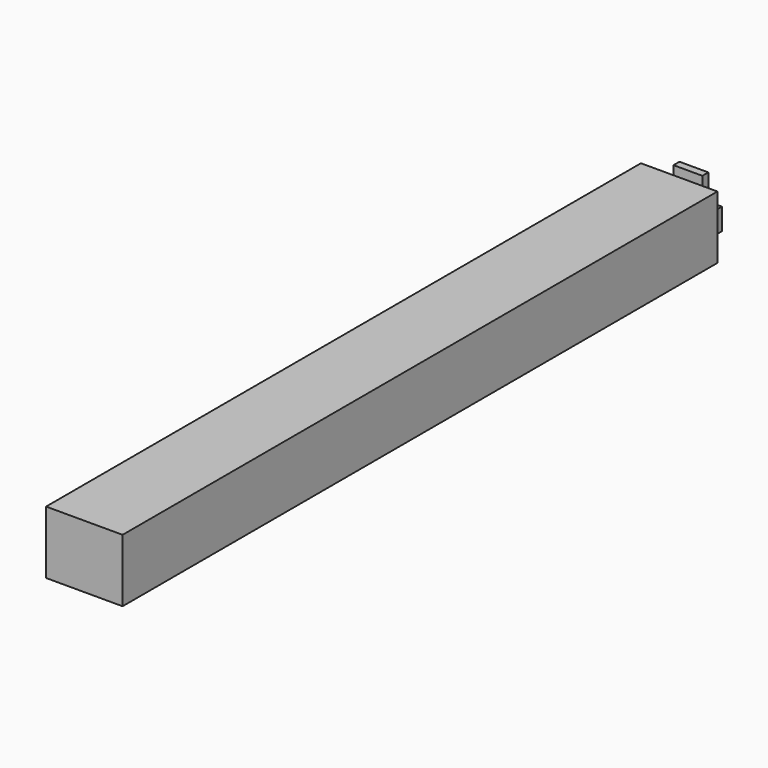
from build123d import *

# Parameters (mm, degrees)
F0_W      = 78.6321908236
F0_H      = 50.2420589328
F0_W_2    = 83.0053240061
F1_DEPTH  = 25.4
F2_W      = 26.6048051417
F2_H      = 12.7
F2_W_2    = 1.4717131853
F2_H_2    = 25.4
F3_DEPTH  = 25.4
F4_W      = 261.3360136747
F4_H      = 214.8963138461
F5_DEPTH  = 2540
F6_W      = 91.9215381145
F6_H      = 68.2068861365
F7_DEPTH  = 25.4
F8_W      = 18.1767717004
F8_H      = 111.8716299534
F8_H_2    = 16.7573786616
F9_DEPTH  = 25.4
F10_W     = 19.8279470205
F10_H     = 1.2968182564
F11_DEPTH = 25.4
F10_W_2   = 29.5902959347
F10_H_2   = 243.1764304638
F12_W     = 25.4
F12_H     = 71.0515528917
F13_DEPTH = 25.4
F14_W     = 21.7962116003
F14_H     = 10.9980255365
F15_DEPTH = 25.4
F16_W     = 95.2623337507
F16_H     = 72.595404768
F17_DEPTH = 25.4
F18_W     = 88.901007548
F18_H     = 12.7
F19_DEPTH = 25.4
F20_W     = 343.005374074
F20_H     = 14.3458449006
F21_DEPTH = 25.4
F22_W     = 127.9820352793
F22_H     = 85.2384865284
F23_DEPTH = 25.4
F24_W     = 127.9820352793
F24_H     = 73.9392116666
F25_DEPTH = 25.4


with BuildPart() as f1:
    # F0 (on Front) → F1 (new body)
    with BuildSketch(Plane.XZ):
        Polygon((-83.0053240061, 0), (0, 0), (78.6321908236, 0), (78.6321908236, 52.9869496822), (-83.0053240061, 52.9869496822), align=None)
        with Locations((39.3160954118, -25.1210294664)):
            Rectangle(F0_W, F0_H)
        with Locations((-41.502662003, -25.1210294664)):
            Rectangle(F0_W_2, F0_H)
    extrude(amount=F1_DEPTH)

    # F2 (on face) → F3 (join)
    with BuildSketch(Plane(origin=(0, 0, -50.2420589328), x_dir=(1, 0, 0), z_dir=(0, 0, -1))):
        Polygon((78.6321908236, 25.7508095026), (-56.4005188644, 25.7508095026), (-56.4005188644, 25.4), (77.1604776382, 25.4), (78.6321908236, 25.4), align=None)
        Polygon((77.1604776382, 25.4), (-56.4005188644, 25.4), (-56.4005188644, 12.7), (-56.4005188644, 0), (77.1604776382, 0), align=None)
        with Locations((-69.7029214352, 19.05)):
            Rectangle(F2_W, F2_H)
        with Locations((77.8963342309, 12.7)):
            Rectangle(F2_W_2, F2_H_2)
        with Locations((-69.7029214352, 6.35)):
            Rectangle(F2_W, F2_H)
    extrude(amount=F3_DEPTH)

    # F4 (on face) → F5 (join)
    with BuildSketch(Plane.XZ.offset(25.4)):
        with Locations((-6.4808502793, -16.0813815892)):
            Rectangle(F4_W, F4_H)
    extrude(amount=F5_DEPTH)

    # F16 (on face) → F17 (join)
    with BuildSketch(Plane(origin=(0, 0, -75.6420589328), x_dir=(1, 0, 0), z_dir=(0, 0, -1))):
        with Locations((-26.4344289899, -10.897702384)):
            Rectangle(F16_W, F16_H)
    extrude(amount=F17_DEPTH)


with BuildPart() as f7:
    # F6 (on face) → F7 (new body)
    with BuildSketch(Plane(origin=(-83.0053240061, 0, 0), x_dir=(0, -1, 0), z_dir=(-1, 0, 0))):
        with Locations((-45.9607690573, -41.5386158645)):
            Rectangle(F6_W, F6_H)
    extrude(amount=F7_DEPTH)


with BuildPart() as f9:
    # F8 (on face) → F9 (new body)
    with BuildSketch(Plane(origin=(-83.0053240061, 0, 0), x_dir=(0, -1, 0), z_dir=(-1, 0, 0))):
        with Locations((9.0883858502, -2.9488652945)):
            Rectangle(F8_W, F8_H)
        with Locations((9.0883858502, -67.263369602)):
            Rectangle(F8_W, F8_H_2)
        Polygon((18.1767717004, 52.9869496822), (18.1767717004, -58.8846802711), (18.1767717004, -75.6420589328), (25.4, -75.6420589328), (25.4, 52.9869496822), align=None)
    extrude(amount=F9_DEPTH)


with BuildPart() as f11:
    # F10 (on face) → F11 (new body)
    with BuildSketch(Plane(origin=(0, 0, 0), x_dir=(-1, 0, 0), z_dir=(0, 1, 0))):
        with Locations((68.9010545611, -190.8378899097)):
            Rectangle(F10_W, F10_H)
    extrude(amount=F11_DEPTH)


with BuildPart() as f11b:
    # F10 (on face) → F11, piece 2 (new body)
    with BuildSketch(Plane(origin=(0, 0, 0), x_dir=(-1, 0, 0), z_dir=(0, 1, 0))):
        with Locations((93.6101760387, -68.6012655497)):
            Rectangle(F10_W_2, F10_H_2)
    extrude(amount=F11_DEPTH)


with BuildPart() as f13:
    # F12 (on face) → F13 (new body)
    with BuildSketch(Plane.XY.offset(-7.4351727962)):
        with Locations((-95.7053240061, 56.3957616687)):
            Rectangle(F12_W, F12_H)
    extrude(amount=F13_DEPTH)


with BuildPart() as f15:
    # F14 (on face) → F15 (new body)
    with BuildSketch(Plane(origin=(0, 0, 0), x_dir=(-1, 0, 0), z_dir=(0, 1, 0))):
        Polygon((78.4667208791, -69.5268400013), (78.4667208791, -80.9810757637), (78.4703195095, -80.9810757637), (100.2665311098, -80.9810757637), (101.8273606896, -80.9810757637), (101.8273606896, -69.5268400013), align=None)
        with Locations((89.3684253097, -86.480088532)):
            Rectangle(F14_W, F14_H)
    extrude(amount=F15_DEPTH)


with BuildPart() as f19:
    # F18 (on face) → F19 (new body)
    with BuildSketch(Plane(origin=(0, 47.195404768, 0), x_dir=(-1, 0, 0), z_dir=(0, 1, 0))):
        with Locations((29.6150920913, -94.6920589328)):
            Rectangle(F18_W, F18_H)
        Polygon((-14.8354116827, -88.3420589328), (74.0655958652, -88.3420589328), (83.8160216808, -88.3420589328), (83.8160216808, 73.4404921532), (-14.8354116827, 73.4404921532), align=None)
    extrude(amount=F19_DEPTH)


with BuildPart() as f21:
    # F20 (on face) → F21 (new body)
    with BuildSketch(Plane(origin=(0, 0, 0), x_dir=(-1, 0, 0), z_dir=(0, 1, 0))):
        with Locations((92.8704962134, -82.8149813831)):
            Rectangle(F20_W, F20_H)
    extrude(amount=F21_DEPTH)


with BuildPart() as f23:
    # F22 (on face) → F23 (new body)
    with BuildSketch(Plane(origin=(0, 0, 0), x_dir=(-1, 0, 0), z_dir=(0, 1, 0))):
        with Locations((-14.6411731839, -42.6192432642)):
            Rectangle(F22_W, F22_H)
    extrude(amount=F23_DEPTH)


with BuildPart() as f25:
    # F24 (on face) → F25 (new body)
    with BuildSketch(Plane(origin=(0, 25.4, 0), x_dir=(-1, 0, 0), z_dir=(0, 1, 0))):
        with Locations((-14.6411731839, -36.9696058333)):
            Rectangle(F24_W, F24_H)
    extrude(amount=F25_DEPTH)


solid = Compound([f1.part, f7.part, f9.part, f11.part, f11b.part, f13.part, f15.part, f19.part, f21.part, f23.part, f25.part])
